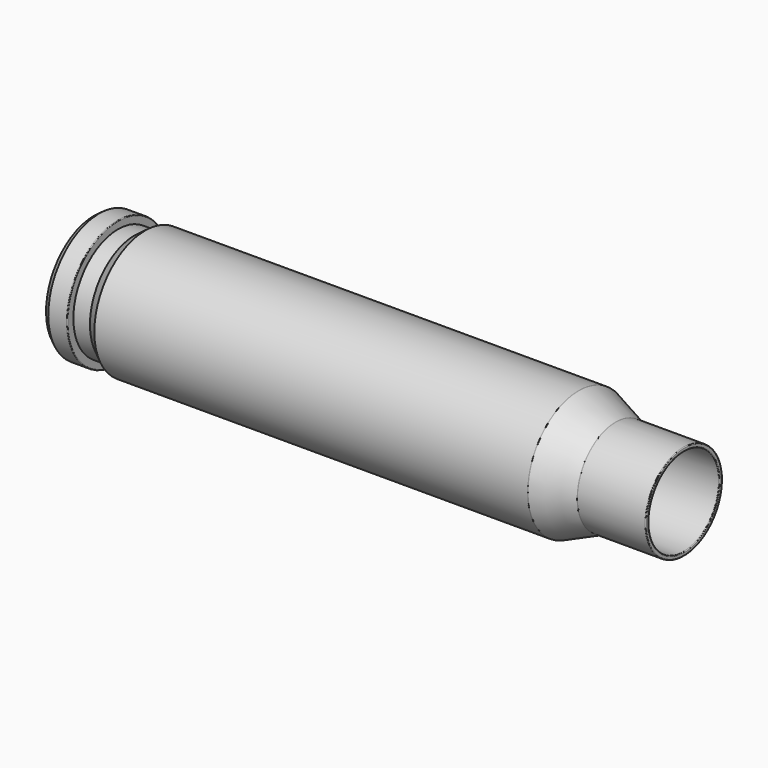
from build123d import *

# Parameters (mm, degrees)
F3_R           = 2.1971
F3_R_2         = 0.73279
F4_DEPTH       = 1.3462
F5_DEPTH       = 4.064
F6_SIZE        = 0.127
F7_R           = 0.0508
F8_R           = 0.0508
F9_TEXT_SIZE   = 1.1880435577
F9_TEXT_SIZE_2 = 1.2550957381
F10_DEPTH      = 0.127
F11_R          = 0.0508


# Not quite as in the source:
# - Text() gives the source's letters only with a copy of the font that has no kerning and outlines rounded to 1/6400 em; it was checked with that copy


with BuildPart() as f2:
    # F0 (on Front) → F2 (revolve)
    with BuildSketch(Plane.XZ):
        Polygon((-35.8992229119, 4.5211209279), (-35.8992229119, 0), (-32.0485829119, 0), (-32.0485829119, 4.064), (0.6259770881, 4.5085), (3.4082950581, 3.327476091), (8.5644950581, 3.327476091), (8.5644950581, 3.606876091), (3.4082950581, 3.606876091), (0.6259770881, 4.7879), (-32.0485829119, 4.7879), (-32.8351851795, 4.2164), (-34.0862464676, 4.2164), (-34.0862464676, 4.7879), (-35.5182229119, 4.7879), align=None)
    revolve(axis=Axis((-0.4805363715, 0, 0), (1, 0, 0)))

    # F3 (on face) → F4 (cut)
    with BuildSketch(Plane(origin=(-35.8992229119, 0, 0), x_dir=(0, -1, 0), z_dir=(-1, 0, 0))):
        Circle(F3_R)
        Circle(F3_R_2, mode=Mode.SUBTRACT)
    extrude(amount=-F4_DEPTH, mode=Mode.SUBTRACT)

    # F5 (cut): a face of the model
    f5_faces = [f2.faces().sort_by_distance(p)[0] for p in [
        (-35.8992229119, 0, 0),
    ]]
    extrude(f5_faces, amount=-F5_DEPTH, mode=Mode.SUBTRACT)

    # F6
    f6_edges = [f2.edges().sort_by_distance(p)[0] for p in [
        (-35.899223, 2.1971, 0),
        (-34.553023, 0.73279, 0),
        (-33.300803, -0.73279, 0),
        (-32.048583, 0.73279, 0),
    ]]
    chamfer(f6_edges, length=F6_SIZE)

    # F7
    f7_edges = [f2.edges().sort_by_distance(p)[0] for p in [
        (0.625977, 0, -4.7879),
        (3.408295, 0, -3.606876),
    ]]
    fillet(f7_edges, radius=F7_R)

    # F8
    f8_edges = [f2.edges().sort_by_distance(p)[0] for p in [
        (-32.048583, 0, -4.7879),
        (-34.086246, 0, -4.7879),
        (-35.518223, 0, -4.7879),
    ]]
    fillet(f8_edges, radius=F8_R)

    # F9 (on face) → F10 (cut)
    with BuildSketch(Plane(origin=(-35.8992229119, 0, 0), x_dir=(0, -1, 0), z_dir=(-1, 0, 0))):
        with Locations((-1.2830865077, 2.8668967659)):
            Text('REM', F9_TEXT_SIZE, font='Open Sans', font_style=FontStyle.BOLD, text_align=(TextAlign.LEFT, TextAlign.BOTTOM))
        with Locations((-1.3499139401, -3.4898904542)):
            Text('.223', F9_TEXT_SIZE_2, font='Open Sans', font_style=FontStyle.BOLD, text_align=(TextAlign.LEFT, TextAlign.BOTTOM))
    extrude(amount=-F10_DEPTH, mode=Mode.SUBTRACT)

    # F11
    f11_edges = [f2.edges().sort_by_distance(p)[0] for p in [
        (8.564495, 0, -3.606876),
        (8.564495, 0, -3.327476),
    ]]
    fillet(f11_edges, radius=F11_R)


solid = f2.part
